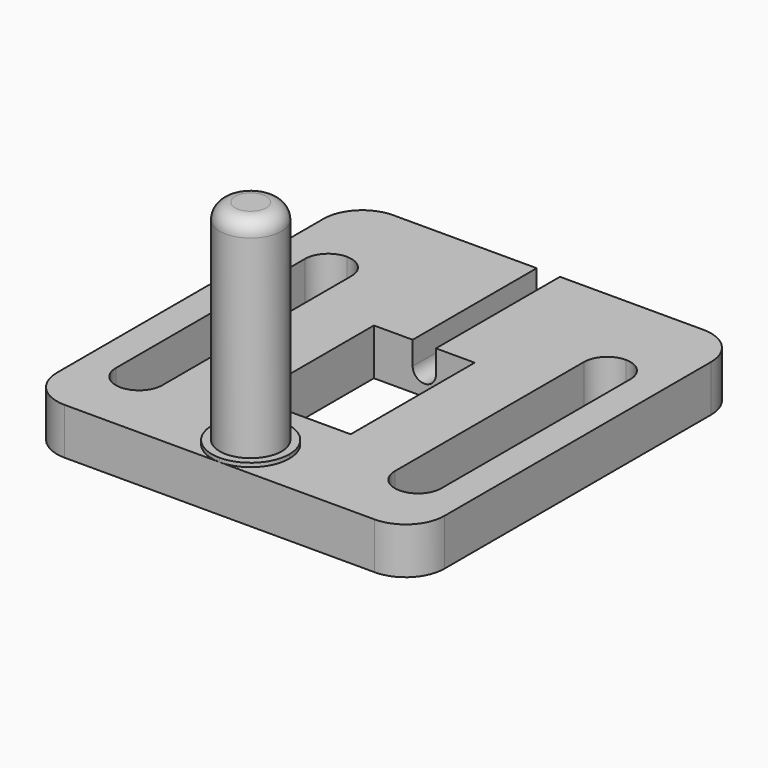
from build123d import *

# Parameters (mm, degrees)
F0_W     = 13
F0_H     = 20
F0_R     = 4
F0_W_2   = 6
F0_H_2   = 3.5
F1_DEPTH = 6
F2_DEPTH = 0.5
F3_R     = 4
F4_DEPTH = 27
F5_R     = 2
F7_DEPTH = 20
F8_R     = 5
F9_R     = 2.99999


# Not quite as in the source:
# - a fillet or chamfer is up to 0.001 mm smaller than in the source, because OpenCascade refuses the exact size


with BuildPart() as f1:
    # F0 (on Top) → F1 (new body)
    with BuildSketch(Plane.XY):
        Polygon((25, 75), (-25, 75), (-25, 22), (0, 22), (25, 22), align=None)
        Polygon((-21, 28.5), (-21, 65), (-15, 65), (-15, 28.5), (-15, 25), (-21, 25), align=None, mode=Mode.SUBTRACT)
        with BuildLine():
            ThreePointArc((5, 27), (3.5355339059, 23.4644660941), (0, 22))
            ThreePointArc((0, 22), (-3.5355339059, 30.5355339059), (5, 27))
        make_face(mode=Mode.SUBTRACT)
        with Locations((0, 45)):
            Rectangle(F0_W, F0_H, mode=Mode.SUBTRACT)
        Polygon((21, 25), (15, 25), (15, 28.5), (15, 65), (21, 65), (21, 28.5), align=None, mode=Mode.SUBTRACT)
        with BuildLine():
            ThreePointArc((5, 27), (-3.5355339059, 30.5355339059), (0, 22))
            ThreePointArc((0, 22), (3.5355339059, 23.4644660941), (5, 27))
        make_face()
        with Locations((0, 27)):
            Circle(F0_R, mode=Mode.SUBTRACT)
        with Locations((0, 27)):
            Circle(F0_R)
        with Locations((18, 26.75)):
            Rectangle(F0_W_2, F0_H_2)
        with Locations((-18, 26.75)):
            Rectangle(F0_W_2, F0_H_2)
    extrude(amount=-F1_DEPTH)

    # F0 (on Top) → F2 (join)
    with BuildSketch(Plane.XY):
        with BuildLine():
            ThreePointArc((5, 27), (-3.5355339059, 30.5355339059), (0, 22))
            ThreePointArc((0, 22), (3.5355339059, 23.4644660941), (5, 27))
        make_face()
        with Locations((0, 27)):
            Circle(F0_R, mode=Mode.SUBTRACT)
        with Locations((0, 27)):
            Circle(F0_R)
    extrude(amount=F2_DEPTH)

    # F3 (on face) → F4 (join)
    with BuildSketch(Plane.XY.offset(0.5)):
        with Locations((0, 27)):
            Circle(F3_R)
    extrude(amount=F4_DEPTH)

    # F5
    f5_edges = [f1.edges().sort_by_distance(p)[0] for p in [
        (-4, 27, 27.5),
    ]]
    fillet(f5_edges, radius=F5_R)

    # F6 (on face) → F7 (cut, through all)
    with BuildSketch(Plane(origin=(0, 75, 0), x_dir=(-1, 0, 0), z_dir=(0, 1, 0))):
        with BuildLine():
            ThreePointArc((-1.5, -3), (0, -4.5), (1.5, -3))
            ThreePointArc((1.5, -3), (0, -1.5), (-1.5, -3))
        make_face()
        with BuildLine():
            ThreePointArc((-1.5, -3), (0, -1.5), (1.5, -3))
            Line((1.5, -3), (1.5, 0))
            Line((1.5, 0), (-1.5, 0))
            Line((-1.5, 0), (-1.5, -3))
        make_face()
    extrude(amount=-F7_DEPTH, mode=Mode.SUBTRACT)

    # F8
    f8_edges = [f1.edges().sort_by_distance(p)[0] for p in [
        (25, 75, -3),
        (-25, 75, -3),
        (-25, 22, -3),
        (25, 22, -3),
    ]]
    fillet(f8_edges, radius=F8_R)

    # F9 (radius 3 in the source; OpenCascade refuses exactly that, so slightly less here)
    f9_edges = [f1.edges().sort_by_distance(p)[0] for p in [
        (-15, 28.5, -3),
        (-21, 28.5, -3),
        (21, 28.5, -3),
        (15, 28.5, -3),
        (21, 65, -3),
        (-15, 65, -3),
        (-21, 65, -3),
        (15, 65, -3),
    ]]
    fillet(f9_edges, radius=F9_R)


solid = f1.part
